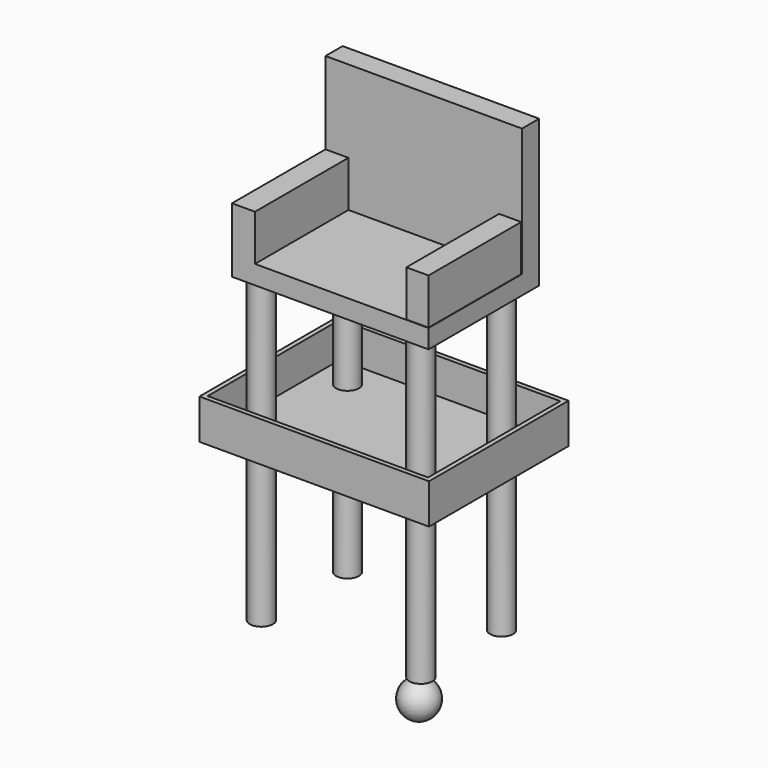
from build123d import *

# Parameters (mm, degrees)
F0_W      = 127
F0_H      = 96.52
F1_DEPTH  = 20.574
F2_T      = -2.54
F4_DEPTH  = 22.098
F5_T      = -2.54
F3_R      = 6.35
F6_DEPTH  = 88.9
F7_DEPTH  = 88.9
F8_W      = 108.7356284261
F8_H      = 76.4898918569
F8_R      = 6.35
F9_DEPTH  = 10.414
F10_W     = 108.7356284261
F10_H     = 11.8554327637
F11_DEPTH = 70.866
F12_W     = 12.7
F12_H     = 64.6344590932
F14_DEPTH = 25.4
F15_W     = 12.2384615242
F15_H     = 64.1062222421
F16_DEPTH = 25.4


with BuildPart() as f1:
    # F0 (on Top) → F1 (new body)
    with BuildSketch(Plane.XY):
        with Locations((4.3395217508, -1.8305095133)):
            Rectangle(F0_W, F0_H)
    extrude(amount=F1_DEPTH)

    # F2
    f2_openings = [f1.faces().sort_by_distance(p)[0] for p in [
        (4.339522, -1.83051, 20.574),
    ]]
    offset(amount=F2_T, openings=f2_openings)


with BuildPart() as f4:
    # F0 (on Top) → F4 (new body)
    with BuildSketch(Plane.XY):
        with Locations((4.3395217508, -1.8305095133)):
            Rectangle(F0_W, F0_H)
    extrude(amount=F4_DEPTH)

    # F5
    f5_openings = [f4.faces().sort_by_distance(p)[0] for p in [
        (4.339522, -1.83051, 22.098),
    ]]
    offset(amount=F5_T, openings=f5_openings)

    # F3 (on face) → F6 (join, symmetric)
    with BuildSketch(Plane(origin=(0, 0, 0), x_dir=(1, 0, 0), z_dir=(0, 0, -1))):
        with Locations((46.3898666203, 28.8518834859)):
            Circle(F3_R)
    extrude(amount=F6_DEPTH, both=True)

    # F3 (on face) → F7 (join, symmetric)
    with BuildSketch(Plane(origin=(0, 0, 0), x_dir=(1, 0, 0), z_dir=(0, 0, -1))):
        with Locations((-40.8363677561, 30.1761776209)):
            Circle(F3_R)
        with Locations((45.9722205997, -27.4009481072)):
            Circle(F3_R)
        with Locations((-39.950568229, -28.2867494971)):
            Circle(F3_R)
    extrude(amount=F7_DEPTH, both=True)

    # F8 (on face) → F9 (join)
    with BuildSketch(Plane.XY.offset(88.9)):
        with Locations((3.918632865, -0.2094898373)):
            Rectangle(F8_W, F8_H)
        with Locations((-39.950568229, 28.2867494971)):
            Circle(F8_R, mode=Mode.SUBTRACT)
    extrude(amount=-F9_DEPTH)

    # F10 (on face) → F11 (join)
    with BuildSketch(Plane.XY.offset(88.9)):
        with Locations((3.918632865, 32.1077397093)):
            Rectangle(F10_W, F10_H)
    extrude(amount=F11_DEPTH)

    # F12 (on face) → F14 (join)
    with BuildSketch(Plane.XY.offset(88.9)):
        with Locations((-44.0991813481, -6.1372062191)):
            Rectangle(F12_W, F12_H)
    extrude(amount=F14_DEPTH)

    # F15 (on face) → F16 (join)
    with BuildSketch(Plane.XY.offset(88.9)):
        with Locations((51.9376751035, -6.1372090131)):
            Rectangle(F15_W, F15_H)
    extrude(amount=F16_DEPTH)


with BuildPart() as f19:
    # F18 (on offset) → F19 (revolve)
    with BuildSketch(Plane.XZ.offset(29.718)):
        with BuildLine():
            ThreePointArc((46.0341759026, -88.9073684812), (36.0330767575, -99.1039108485), (46.0341759026, -109.3004532158))
            Line((46.0341759026, -109.3004532158), (46.0341759026, -88.9073684812))
        make_face()
    revolve(axis=Axis((46.0341759026, -29.718, -99.1039108485), (0, 0, 1)))


solid = Compound([f1.part, f4.part, f19.part])
